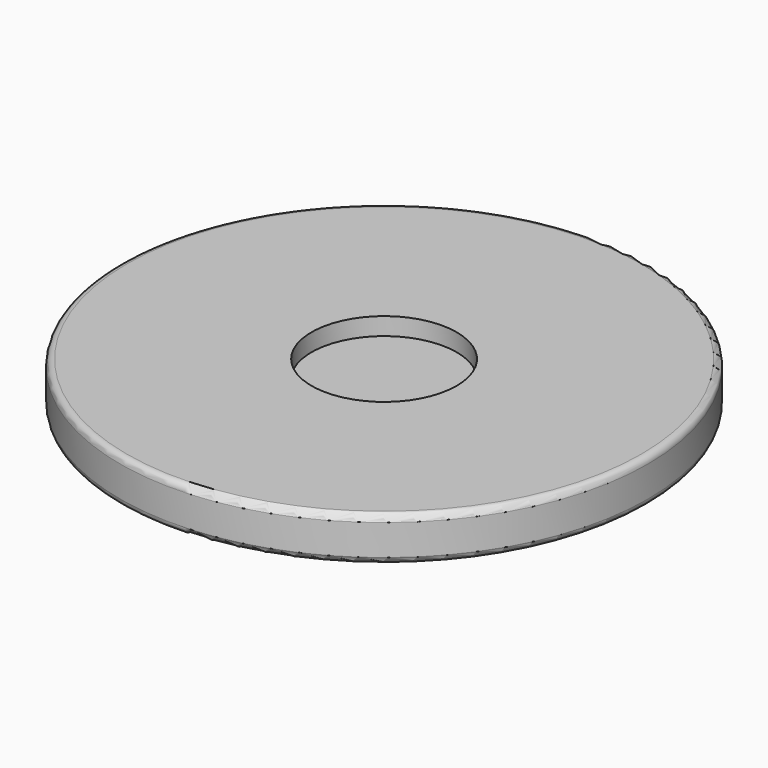
from build123d import *

# Parameters (mm, degrees)
F0_R     = 6
F1_DEPTH = 1
F2_R     = 0.15
F3_R     = 1.65
F4_DEPTH = 0.4


# Not quite as in the source:
# - a feature names something its author has since deleted; it is built from what else it names


with BuildPart() as f1:
    # F0 (on Top) → F1 (new body)
    with BuildSketch(Plane.XY):
        Circle(F0_R)
    extrude(amount=F1_DEPTH)

    # F2
    f2_edges = [f1.edges().sort_by_distance(p)[0] for p in [
        (-6, 0, 1),
        (-6, 0, 0),
    ]]
    fillet(f2_edges, radius=F2_R)

    # F3 (on face) → F4 (cut)
    with BuildSketch(Plane.XY.offset(1)):
        Circle(F3_R)
    extrude(amount=-F4_DEPTH, mode=Mode.SUBTRACT)


solid = f1.part
